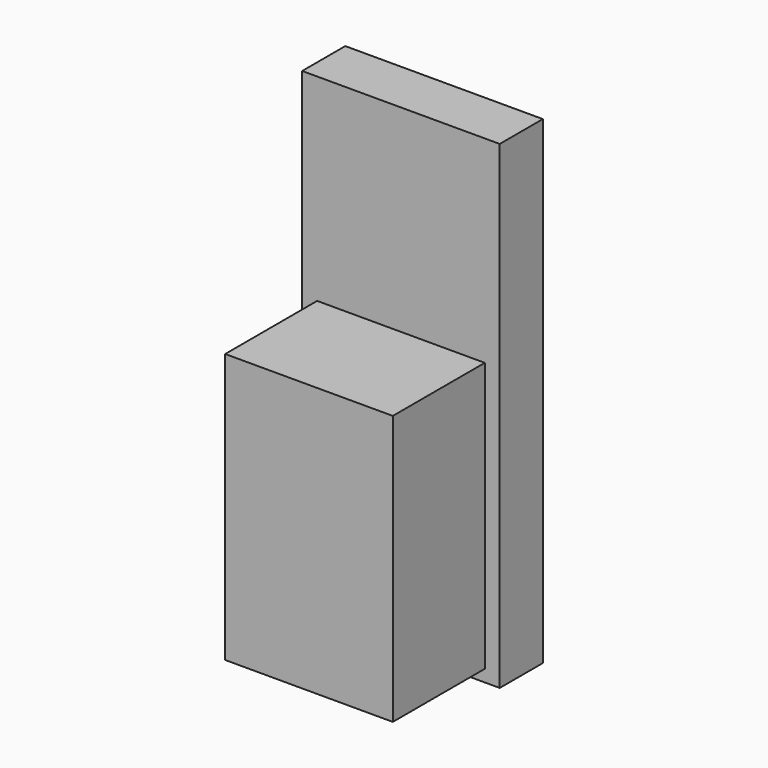
from build123d import *

# Parameters (mm, degrees)
F0_W     = 96
F0_H     = 225
F1_DEPTH = 70
F2_DEPTH = 82.5


# Not quite as in the source:
# - a feature names something its author has since deleted; it is built from what else it names


with BuildPart() as f1:
    # F0 (on Right) → F1 (new body, symmetric)
    with BuildSketch(Plane.YZ):
        with Locations((-70.5, -77.5)):
            Rectangle(F0_W, F0_H)
    extrude(amount=F1_DEPTH, both=True)


with BuildPart() as f2:
    # F0 (on Right) → F2 (new body, symmetric)
    with BuildSketch(Plane.YZ):
        Polygon((-22.5, -190), (-22.5, -200), (22.5, -200), (22.5, 200), (-22.5, 200), (-22.5, 35), align=None)
    extrude(amount=F2_DEPTH, both=True)


solid = Compound([f1.part, f2.part])
